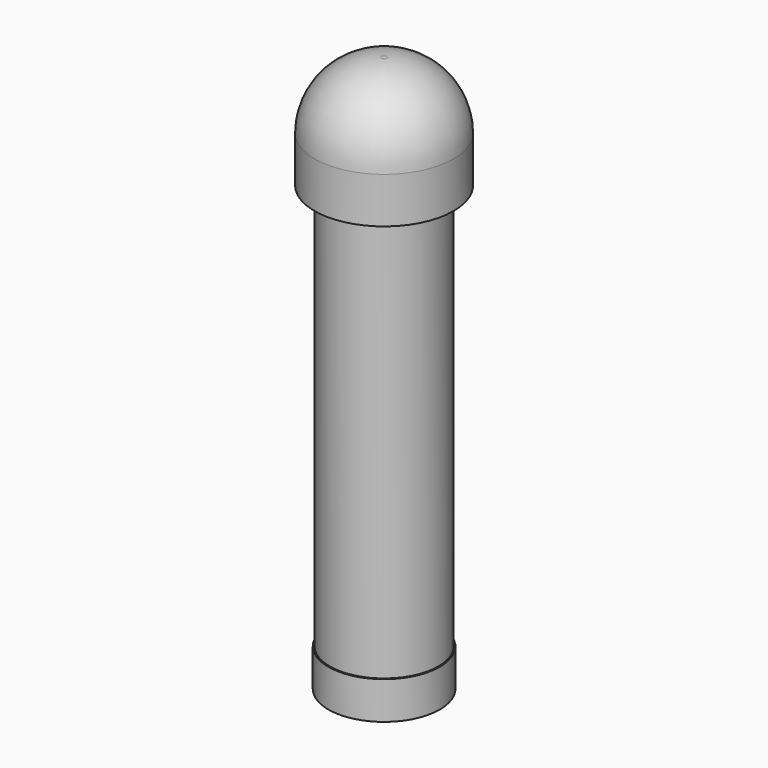
from build123d import *

# Parameters (mm, degrees)
F0_R     = 1.8369282596
F1_DEPTH = 13.716
F2_R     = 2.3492385246
F3_DEPTH = 3.81
F4_R     = 2.2606
F5_R     = 1.8828271996
F5_R_2   = 1.8369282596
F6_DEPTH = 1.27


with BuildPart() as f1:
    # F0 (on Top) → F1 (new body)
    with BuildSketch(Plane.XY):
        Circle(F0_R)
    extrude(amount=F1_DEPTH)


with BuildPart() as f3:
    # F2 (on face) → F3 (new body)
    with BuildSketch(Plane.XY.offset(13.716)):
        Circle(F2_R)
    extrude(amount=F3_DEPTH)

    # F4
    f4_edges = [f3.edges().sort_by_distance(p)[0] for p in [
        (-2.349239, 0, 17.526),
    ]]
    fillet(f4_edges, radius=F4_R)


with BuildPart() as f6:
    # F5 (on face) → F6 (new body)
    with BuildSketch(Plane(origin=(0, 0, 0), x_dir=(1, 0, 0), z_dir=(0, 0, -1))):
        Circle(F5_R)
        Circle(F5_R_2, mode=Mode.SUBTRACT)
        Circle(F5_R_2)
    extrude(amount=F6_DEPTH)


solid = Compound([f1.part, f3.part, f6.part])
